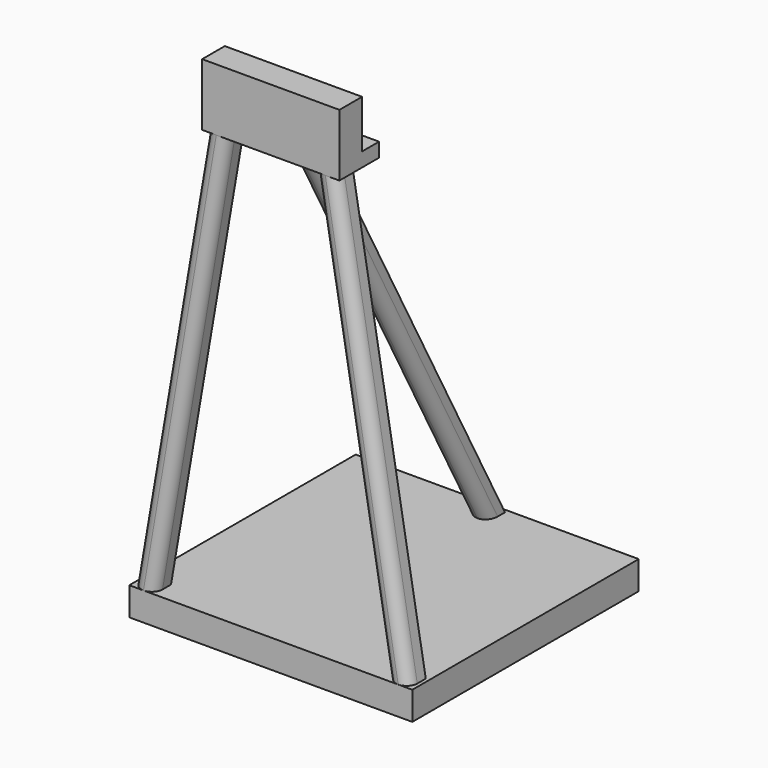
from build123d import *

# Parameters (mm, degrees)
F0_W           = 200
F0_H           = 200
F1_DEPTH       = 10
F2_W           = 20
F2_H           = 34
F3_DEPTH       = 48.5
F5_W           = 15
F5_H           = 15
F11_F1_R       = 7.5
F11_F2_R       = 7.4999
F11_2_T1_DEPTH = 341.8883210637
F11_2_T3_DEPTH = 341.8883210637
F11_3_T1_DEPTH = 341.8883210637
F11_3_T3_DEPTH = 341.8883210637


# Not quite as in the source:
# - a fillet or chamfer that OpenCascade refuses, or shapes differently, is made with other operations: its cross-section is extruded or revolved along the edge and cut away or added
# - a fillet or chamfer is up to 0.001 mm smaller than in the source, because OpenCascade refuses the exact size


with BuildPart() as f1:
    # F0 (on Top) → F1 (new body, symmetric)
    with BuildSketch(Plane.XY):
        Rectangle(F0_W, F0_H)
    extrude(amount=F1_DEPTH, both=True)


with BuildPart() as f3:
    # F2 (on Right) → F3 (new body, symmetric)
    with BuildSketch(Plane.YZ):
        Polygon((15, 0), (0, 0), (-20, 0), (-20, -10), (15, -10), align=None)
        with Locations((-10, 17)):
            Rectangle(F2_W, F2_H)
    extrude(amount=F3_DEPTH, both=True)


with BuildPart() as f3_1:
    # F4: moved
    add(f3.part.moved(Location((0, -80, 320))))


with BuildPart() as f7:
    # F7: sweep along a path in F6
    with BuildLine(Plane.XZ.offset(100)) as f7_path:
        Line((-38.5, 310), (-90, 10))
    # F5 (on face) → F7 (sweep)
    with BuildSketch(Plane(origin=(0, 0, 310), x_dir=(1, 0, 0), z_dir=(0, 0, -1))):
        with Locations((-38.5, 92.5)):
            Rectangle(F5_W, F5_H)
    sweep(path=f7_path.line)

    # F11#2: fillet of radius 7.5 on 2 edges, made by hand

    # F11_2_s2 → F11_2_t1 (cut)
    with BuildSketch(Plane(origin=(53.9782382244, 0, 314.4363391713), x_dir=(0, 1, 0), z_dir=(-0.1691917739, 0, -0.985583149))):
        with BuildLine():
            ThreePointArc((-92.5, -83.0025275336), (-97.8033008589, -85.1992266747), (-100, -90.5025275336))
            Line((-100, -90.5025275336), (-100, -83.0025275336))
            Line((-100, -83.0025275336), (-92.5, -83.0025275336))
        make_face()
    extrude(amount=F11_2_T1_DEPTH, mode=Mode.SUBTRACT)

    # F11_2_s4 → F11_2_t3 (cut)
    with BuildSketch(Plane(origin=(53.548850379, 0, 311.9350507514), x_dir=(0, 1, 0), z_dir=(-0.1691917739, 0, -0.985583149))):
        with BuildLine():
            ThreePointArc((-100, -90.286274769), (-97.8033008589, -95.5895756279), (-92.5, -97.786274769))
            Line((-92.5, -97.786274769), (-100, -97.786274769))
            Line((-100, -97.786274769), (-100, -90.286274769))
        make_face()
    extrude(amount=F11_2_T3_DEPTH, mode=Mode.SUBTRACT)


with BuildPart() as f8:
    # F8: sweep along a path in F6
    with BuildLine(Plane.XZ.offset(100)) as f8_path:
        Line((38.5, 310), (90, 10))
    # F5 (on face) → F8 (sweep)
    with BuildSketch(Plane(origin=(0, 0, 310), x_dir=(1, 0, 0), z_dir=(0, 0, -1))):
        with Locations((38.5, 92.5)):
            Rectangle(F5_W, F5_H)
    sweep(path=f8_path.line)

    # F11#3: fillet of radius 7.5 on 2 edges, made by hand

    # F11_3_s2 → F11_3_t1 (cut)
    with BuildSketch(Plane(origin=(-53.548850379, 0, 311.9350507514), x_dir=(0, 1, 0), z_dir=(0.1691917739, 0, -0.985583149))):
        with BuildLine():
            ThreePointArc((-100, 90.286274769), (-97.8033008589, 95.5895756279), (-92.5, 97.786274769))
            Line((-92.5, 97.786274769), (-100, 97.786274769))
            Line((-100, 97.786274769), (-100, 90.286274769))
        make_face()
    extrude(amount=F11_3_T1_DEPTH, mode=Mode.SUBTRACT)

    # F11_3_s4 → F11_3_t3 (cut)
    with BuildSketch(Plane(origin=(-53.9782382244, 0, 314.4363391713), x_dir=(0, 1, 0), z_dir=(0.1691917739, 0, -0.985583149))):
        with BuildLine():
            ThreePointArc((-100, 90.5025275336), (-97.8033008589, 85.1992266747), (-92.5, 83.0025275336))
            Line((-92.5, 83.0025275336), (-100, 83.0025275336))
            Line((-100, 83.0025275336), (-100, 90.5025275336))
        make_face()
    extrude(amount=F11_3_T3_DEPTH, mode=Mode.SUBTRACT)


with BuildPart() as f10:
    # F10: sweep along a path in F9
    with BuildLine(Plane.YZ) as f10_path:
        Line((-72.5, 310), (90, 10))
    # F5 (on face) → F10 (sweep)
    with BuildSketch(Plane(origin=(0, 0, 310), x_dir=(1, 0, 0), z_dir=(0, 0, -1))):
        with Locations((0, 72.5)):
            Rectangle(F5_W, F5_H)
    sweep(path=f10_path.line)

    # F11: fillet of radius 7.5 on 2 edges, made by hand

    # F11_f1
    f11_f1_edges = [f10.edges().sort_by_distance(p)[0] for p in [
        (-7.5, 1.25, 160),
    ]]
    fillet(f11_f1_edges, radius=F11_F1_R)

    # F11_f2 (radius 7.5 in the source; OpenCascade refuses exactly that, so slightly less here)
    f11_f2_edges = [f10.edges().sort_by_distance(p)[0] for p in [
        (7.5, 1.25, 160),
    ]]
    fillet(f11_f2_edges, radius=F11_F2_R)


solid = Compound([f1.part, f3_1.part, f7.part, f8.part, f10.part])
